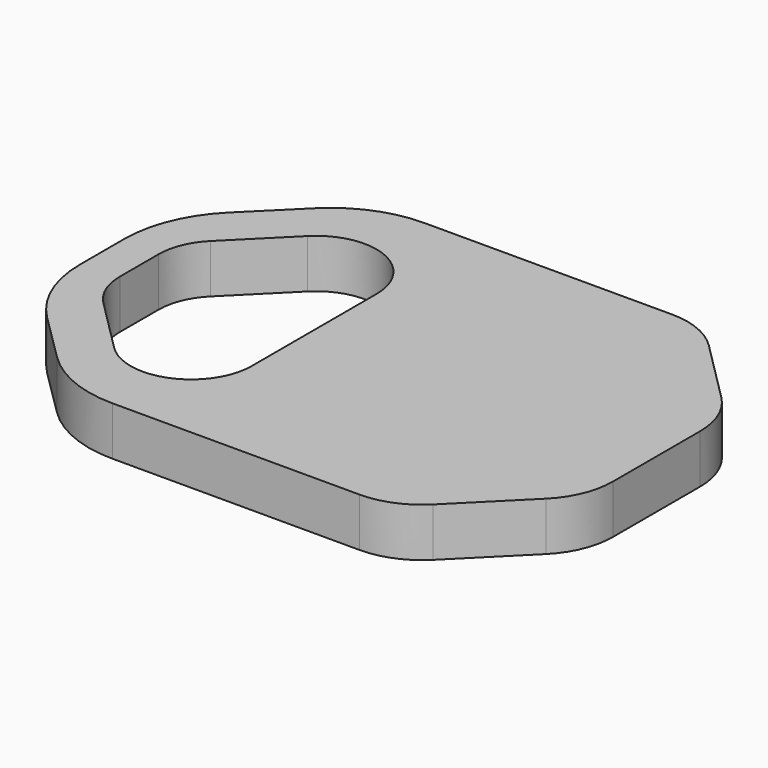
from build123d import *

# Parameters (mm, degrees)
F1_DEPTH = 6.35


# Not quite as in the source:
# - a feature names something its author has since deleted; it is built from what else it names


with BuildPart() as f1:
    # F0 (on Top) → F1 (new body)
    with BuildSketch(Plane.XY):
        with BuildLine():
            ThreePointArc((69.4316146906, -39.8903370424), (71.634025844, -36.5941958184), (72.4074097937, -32.7061321456))
            Line((72.4074097937, -32.7061321456), (72.4074097937, -18.516951733))
            ThreePointArc((72.4074097937, -18.516951733), (71.634025844, -14.6288880601), (69.4316146906, -11.3327468361))
            Line((69.4316146906, -11.3327468361), (61.2862048969, -3.1873370424))
            ThreePointArc((61.2862048969, -3.1873370424), (57.9900636728, -0.9849258889), (54.102, -0.2115419393))
            Line((54.102, -0.2115419393), (21.9140133571, -0.2115419393))
            ThreePointArc((21.9140133571, -0.2115419393), (16.1111416714, -1.3595484607), (11.1825133635, -4.6306127791))
            Line((11.1825133635, -4.6306127791), (4.9301931337, -10.8312609409))
            ThreePointArc((4.9301931337, -10.8312609409), (1.4826892564, -15.9562170355), (0.2714097937, -22.0128877397))
            Line((0.2714097937, -22.0128877397), (0.2714097937, -29.2101961388))
            ThreePointArc((0.2714097937, -29.2101961388), (1.4826892564, -35.266866843), (4.9301931337, -40.3918229376))
            Line((4.9301931337, -40.3918229376), (11.1825133635, -46.5924710994))
            ThreePointArc((11.1825133635, -46.5924710994), (16.1111416714, -49.8635354178), (21.9140133571, -51.0115419393))
            Line((21.9140133571, -51.0115419393), (54.102, -51.0115419393))
            ThreePointArc((54.102, -51.0115419393), (57.9900636728, -50.2381579896), (61.2862048969, -48.0357468361))
            Line((61.2862048969, -48.0357468361), (69.4316146906, -39.8903370424))
        make_face()
        with BuildLine():
            Line((27.8558097937, -15.4515419393), (27.8558097937, -35.7715419393))
            ThreePointArc((27.8558097937, -35.7715419393), (25.5495685888, -41.3393007343), (19.9818097937, -43.6455419393))
            ThreePointArc((19.9818097937, -43.6455419393), (16.9685604473, -43.0461693783), (14.4140509986, -41.3393007343))
            Line((14.4140509986, -41.3393007343), (7.4036509986, -34.3289007343))
            ThreePointArc((7.4036509986, -34.3289007343), (5.6967823547, -31.7743912857), (5.0974097937, -28.7611419393))
            Line((5.0974097937, -28.7611419393), (5.0974097937, -22.4619419393))
            ThreePointArc((5.0974097937, -22.4619419393), (5.6967823547, -19.4486925928), (7.4036509986, -16.8941831442))
            Line((7.4036509986, -16.8941831442), (14.4140509986, -9.8837831442))
            ThreePointArc((14.4140509986, -9.8837831442), (22.9950591402, -8.1769145003), (27.8558097937, -15.4515419393))
        make_face(mode=Mode.SUBTRACT)
    extrude(amount=F1_DEPTH)


solid = f1.part
